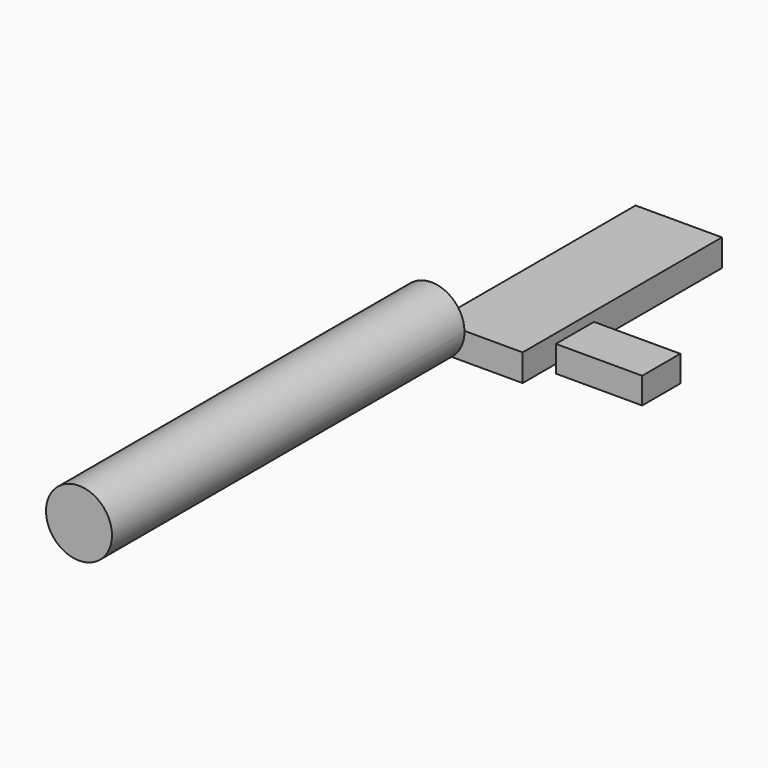
from build123d import *

# Parameters (mm, degrees)
F1_R     = 9.9046935717
F2_DEPTH = 132.334
F4_W     = 25.9259901941
F4_H     = 74.8111829162
F5_DEPTH = 0.254
F6_W     = 25.9226001799
F6_H     = 14.3088037148
F7_DEPTH = 7.874


# Not quite as in the source:
# - the program builds the solid bodies; features that only make, move or delete a surface that nothing else refers to are left out


with BuildPart() as f2:
    # F1 (on Front) → F2 (new body)
    with BuildSketch(Plane.XZ):
        with Locations((-1.4416209888, 0)):
            Circle(F1_R)
    extrude(amount=F2_DEPTH)

    # F4 (on Top) → F5 (join)
    with BuildSketch(Plane.XY):
        with Locations((12.962995097, 37.4055914581)):
            Rectangle(F4_W, F4_H)
    extrude(amount=F5_DEPTH)

    # F6 (on Top) + F5_face (on face) + F5_face1 (on face) → F7 (join)
    with BuildSketch(Plane.XY):
        with Locations((41.966361925, 15.7852205448)):
            Rectangle(F6_W, F6_H)
    with BuildSketch(Plane(origin=(12.962995097, 37.4055914581, 0), x_dir=(1, 0, 0), z_dir=(0, 0, -1))):
        Polygon((-12.962995097, 37.4055914581), (-12.962995097, -37.4055914581), (12.962995097, -37.4055914581), (12.962995097, 37.4055914581), (-4.4999225141, 37.4055914581), align=None)
    with BuildSketch(Plane(origin=(12.962995097, 37.4055914581, 0.254), x_dir=(1, 0, 0), z_dir=(0, 0, 1))):
        Polygon((-12.962995097, 37.4055914581), (-12.962995097, -37.4055914581), (-4.5031798895, -37.4055914581), (12.962995097, -37.4055914581), (12.962995097, 37.4055914581), align=None)
    extrude(amount=-F7_DEPTH, dir=(0, 0, 1))


solid = f2.part
